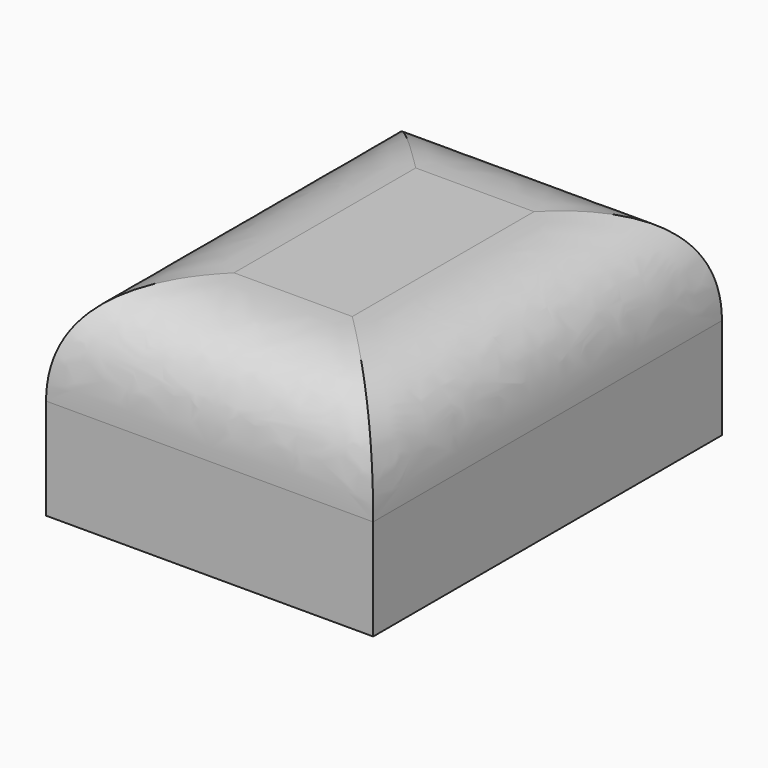
from build123d import *

# Parameters (mm, degrees)
F0_W        = 23.8764360547
F0_H        = 31.8190380931
F3_DEPTH    = 12.7
F1_T1_DEPTH = 69.9190380931
F1_T3_DEPTH = 61.9764360547
F2_DEPTH    = 2.286


# Not quite as in the source:
# - a fillet or chamfer that OpenCascade refuses, or shapes differently, is made with other operations: its cross-section is extruded or revolved along the edge and cut away or added


with BuildPart() as f3:
    # F0 (on Top) → F3 (new body)
    with BuildSketch(Plane.XY):
        with Locations((11.9382180274, -15.9095190465)):
            Rectangle(F0_W, F0_H)
    extrude(amount=F3_DEPTH)

    # F1: fillet of radius 7.62 on 4 edges, made by hand

    # F1_s2 → F1_t1 (cut)
    with BuildSketch(Plane.XZ.offset(-19.05)):
        with BuildLine():
            add(Edge.make_bspline(
                [(23.8764360547, 5.08), (23.8764360547, 12.7), (16.2564360547, 12.7)],
                knots=[0, 0, 0, 1, 1, 1], degree=2, weights=[1, 1, 1]))
            Line((16.2564360547, 12.7), (23.8764360547, 12.7))
            Line((23.8764360547, 12.7), (23.8764360547, 5.08))
        make_face()
        with BuildLine():
            add(Edge.make_bspline(
                [(0, 5.08), (0, 12.7), (7.62, 12.7)],
                knots=[0, 0, 0, 1, 1, 1], degree=2, weights=[1, 1, 1]))
            Line((7.62, 12.7), (0, 12.7))
            Line((0, 12.7), (0, 5.08))
        make_face()
    extrude(amount=F1_T1_DEPTH, mode=Mode.SUBTRACT)

    # F1_s4 → F1_t3 (cut)
    with BuildSketch(Plane.YZ.offset(-19.05)):
        with BuildLine():
            add(Edge.make_bspline(
                [(0, 5.08), (0, 12.7), (-7.62, 12.7)],
                knots=[0, 0, 0, 1, 1, 1], degree=2, weights=[1, 1, 1]))
            Line((-7.62, 12.7), (0, 12.7))
            Line((0, 12.7), (0, 5.08))
        make_face()
        with BuildLine():
            add(Edge.make_bspline(
                [(-31.8190380931, 5.08), (-31.8190380931, 12.7), (-24.1990380931, 12.7)],
                knots=[0, 0, 0, 1, 1, 1], degree=2, weights=[1, 1, 1]))
            Line((-24.1990380931, 12.7), (-31.8190380931, 12.7))
            Line((-31.8190380931, 12.7), (-31.8190380931, 5.08))
        make_face()
    extrude(amount=F1_T3_DEPTH, mode=Mode.SUBTRACT)

    # F2 (add): a face of the model
    f2_faces = [f3.faces().sort_by_distance(p)[0] for p in [
        (11.9382180274, -15.9095190465, 0),
    ]]
    extrude(f2_faces, amount=F2_DEPTH)


solid = f3.part
